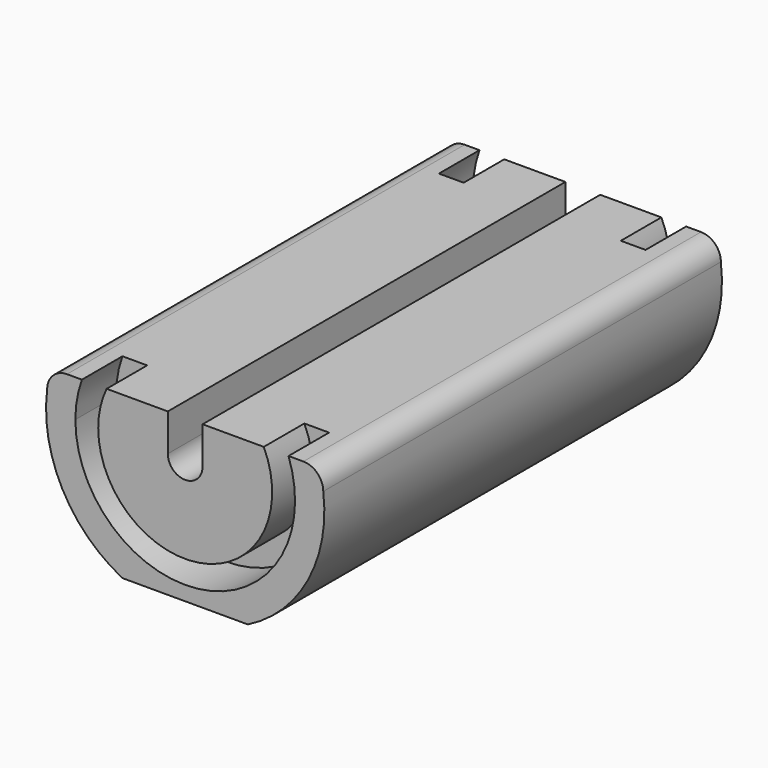
from build123d import *

# Parameters (mm, degrees)
F0_W     = 12.1401943831
F0_H     = 2
F1_DEPTH = 25
F4_DEPTH = 5.1
F8_R     = 1.99999


# Not quite as in the source:
# - a fillet or chamfer is up to 0.001 mm smaller than in the source, because OpenCascade refuses the exact size


with BuildPart() as f1:
    # F0 (on Front) → F1 (new body)
    with BuildSketch(Plane.XZ):
        with BuildLine():
            Line((-1.75, 1.75), (-13.8901943831, 1.75))
            ThreePointArc((-13.8901943831, 1.75), (-12.3581823788, -6.5783986115), (-6.3047601065, -12.5))
            Line((-6.3047601065, -12.5), (6.3047601065, -12.5))
            ThreePointArc((6.3047601065, -12.5), (12.3581823788, -6.5783986115), (13.8901943831, 1.75))
            Line((13.8901943831, 1.75), (1.75, 1.75))
            Line((1.75, 1.75), (1.75, 0))
            ThreePointArc((1.75, 0), (0, -1.75), (-1.75, 0))
            Line((-1.75, 0), (-1.75, 1.75))
        make_face()
        with Locations((7.8200971915, 2.75)):
            Rectangle(F0_W, F0_H)
        with Locations((-7.8200971915, 2.75)):
            Rectangle(F0_W, F0_H)
    extrude(amount=F1_DEPTH)

    # F3 (on face) → F4 (cut)
    with BuildSketch(Plane(origin=(0, 0, 0), x_dir=(-1, 0, 0), z_dir=(0, 1, 0))):
        with BuildLine():
            ThreePointArc((-10.3942291681, 3.75), (-1.9034531373, -10.8848227433), (11.05, 0))
            ThreePointArc((11.05, 0), (10.8848227433, 1.9034531373), (10.3942291681, 3.75))
            Line((10.3942291681, 3.75), (7.9056941504, 3.75))
            ThreePointArc((7.9056941504, 3.75), (8.5363143047, 1.921936027), (8.75, 0))
            ThreePointArc((8.75, 0), (-1.921936027, -8.5363143047), (-7.9056941504, 3.75))
            Line((-7.9056941504, 3.75), (-10.3942291681, 3.75))
        make_face()
    extrude(amount=-F4_DEPTH, mode=Mode.SUBTRACT)

    # F7: F1 across face


with BuildPart() as f1_1:
    add(f1.part)
    add(f1.part.mirror(Plane(origin=(0, -25, -3.8986050214), x_dir=(1, 0, 0), z_dir=(0, -1, 0))))

    # F8 (radius 2 in the source; OpenCascade refuses exactly that, so slightly less here)
    f8_edges = [f1_1.edges().sort_by_distance(p)[0] for p in [
        (13.890194, -25, 3.75),
        (-13.890194, -25, 3.75),
    ]]
    fillet(f8_edges, radius=F8_R)


solid = f1_1.part
